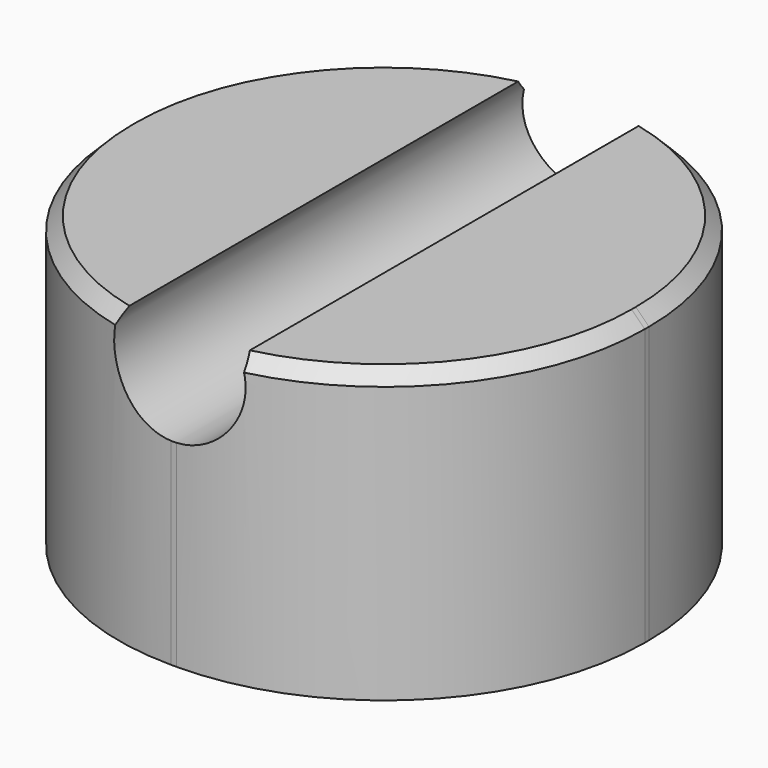
from build123d import *

# Parameters (mm, degrees)
F1_DEPTH     = 6
F2_R         = 2.5
F3_DEPTH     = 25
F4_T1_DEPTH  = 0.2
F4_T4_ANGLE  = 84.656067133
F4_T6_ANGLE  = 84.656067133
F4_T8_ANGLE  = 84.656067133
F4_T10_ANGLE = 84.656067133
F5_DEPTH     = 5


# Not quite as in the source:
# - a fillet or chamfer that OpenCascade refuses, or shapes differently, is made with other operations: its cross-section is extruded or revolved along the edge and cut away or added


with BuildPart() as f1:
    # F0 (on Top) → F1 (new body)
    with BuildSketch(Plane.XY):
        with BuildLine():
            Line((-3.071964772, 10.9479769804), (-3.271964772, 10.9479769804))
            ThreePointArc((-3.271964772, 10.9479769804), (-10.2723219058, 8.0483341141), (-13.171964772, 1.0479769804))
            Line((-13.171964772, 1.0479769804), (-13.171964772, 0.8479769804))
            ThreePointArc((-13.171964772, 0.8479769804), (-10.2723219058, -6.1523801534), (-3.271964772, -9.0520230196))
            Line((-3.271964772, -9.0520230196), (-3.071964772, -9.0520230196))
            ThreePointArc((-3.071964772, -9.0520230196), (3.9283923617, -6.1523801534), (6.828035228, 0.8479769804))
            Line((6.828035228, 0.8479769804), (6.828035228, 1.0479769804))
            ThreePointArc((6.828035228, 1.0479769804), (3.9283923617, 8.0483341141), (-3.071964772, 10.9479769804))
        make_face()
    extrude(amount=F1_DEPTH)

    # F2 (on face) → F3 (cut)
    with BuildSketch(Plane.XZ.offset(9.0520230196)):
        with Locations((-3.171964772, 5)):
            Circle(F2_R)
    extrude(amount=-F3_DEPTH, mode=Mode.SUBTRACT)

    # F4: chamfer of 0.5 on 2 edges, made by hand

    # F4_s2 → F4_t1 (cut)
    with BuildSketch(Plane.XZ.offset(-1.0479769804)):
        Polygon((-13.171964772, 5.5), (-12.671964772, 6), (-13.171964772, 6), align=None)
        Polygon((6.828035228, 5.5), (6.328035228, 6), (6.828035228, 6), align=None)
    extrude(amount=F4_T1_DEPTH, mode=Mode.SUBTRACT)

    # F4_s3 → F4_t4 (revolve, cut)
    with BuildSketch(Plane.XZ.offset(-1.0479769804)):
        Polygon((6.328035228, 6), (6.828035228, 5.5), (6.828035228, 6), align=None)
    revolve(axis=Axis((-3.071964772, 1.0479769804, 6), (0, 0, 1)), revolution_arc=F4_T4_ANGLE, mode=Mode.SUBTRACT)

    # F4_s5 → F4_t6 (revolve, cut)
    with BuildSketch(Plane(origin=(-3.1464057809, -0.2943167545, 0), x_dir=(0, 0, 1), z_dir=(0.9956535782, 0.0931340552, 0))):
        Polygon((5.5, -11.2481533781), (6, -10.7481533781), (6, -11.2481533781), align=None)
    revolve(axis=Axis((-3.271964772, 1.0479769804, 6), (0, 0, 1)), revolution_arc=F4_T6_ANGLE, mode=Mode.SUBTRACT)

    # F4_s7 → F4_t8 (revolve, cut)
    with BuildSketch(Plane.XZ.offset(-0.8479769804)):
        Polygon((-12.671964772, 6), (-13.171964772, 5.5), (-13.171964772, 6), align=None)
    revolve(axis=Axis((-3.271964772, 0.8479769804, 6), (0, 0, 1)), revolution_arc=F4_T8_ANGLE, mode=Mode.SUBTRACT)

    # F4_s9 → F4_t10 (revolve, cut)
    with BuildSketch(Plane(origin=(-2.9666864224, -0.2775056939, 0), x_dir=(0, 0, 1), z_dir=(-0.9956535782, -0.0931340552, 0))):
        Polygon((6, -8.2696041486), (5.5, -8.7696041486), (6, -8.7696041486), align=None)
    revolve(axis=Axis((-3.071964772, 0.8479769804, 6), (0, 0, 1)), revolution_arc=F4_T10_ANGLE, mode=Mode.SUBTRACT)

    # F5 (add): a face of the model
    f5_faces = [f1.faces().sort_by_distance(p)[0] for p in [
        (-3.171964772, 0.9479769804, 0),
    ]]
    extrude(f5_faces, amount=F5_DEPTH)


solid = f1.part
